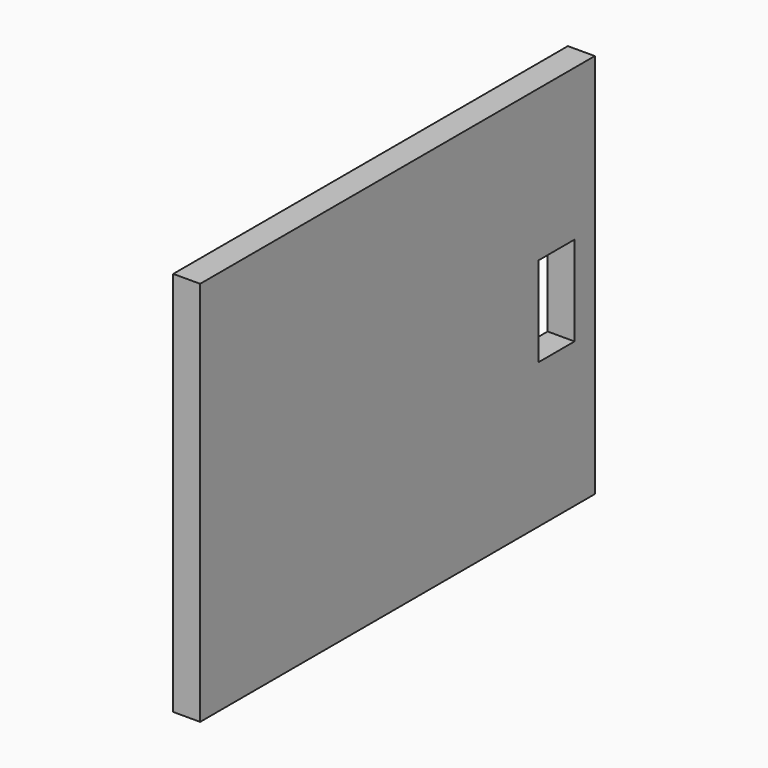
from build123d import *

# Parameters (mm, degrees)
F0_W     = 5.000215
F0_H     = 10.000086
F1_DEPTH = 3


# Not quite as in the source:
# - ends of sketch curves that miss each other by under 0.0002 mm in the source are joined


with BuildPart() as f1:
    # F0 (on Right) → F1 (new body)
    with BuildSketch(Plane.YZ):
        Polygon((-27.499976, 19.999999), (-27.499976, -19.999998), (27.499976, -19.999998), (27.500024, 19.999999), (27.499976, 23.000002), (-27.499976, 23.000002), align=None)
        with Locations((22.1822251524, 1.1325399325)):
            Rectangle(F0_W, F0_H, mode=Mode.SUBTRACT)
    extrude(amount=F1_DEPTH)


solid = f1.part
